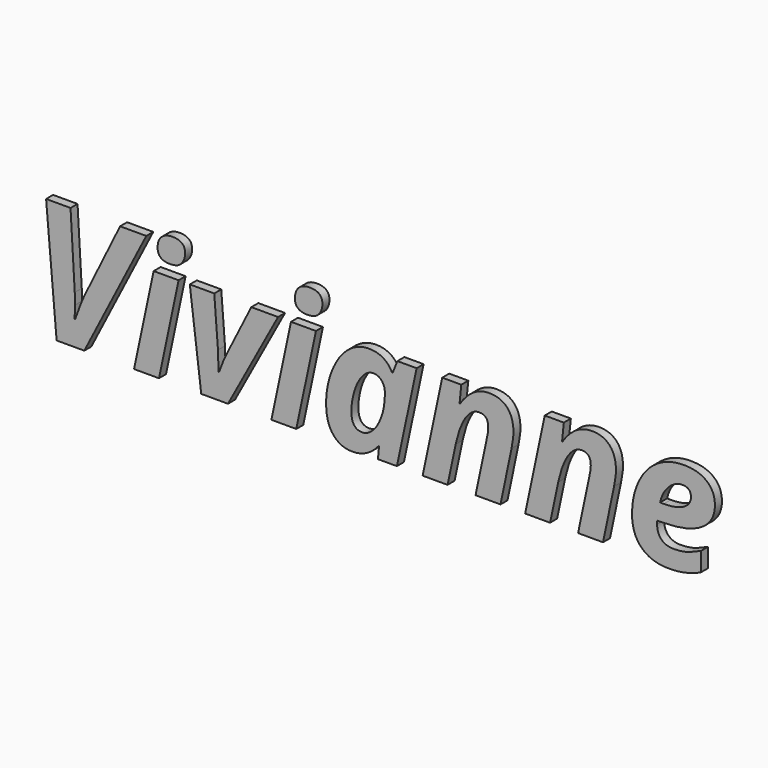
from build123d import *

# Parameters (mm, degrees)
F0_TEXT_SIZE = 61.4441750157
F1_DEPTH     = 3.175


# Not quite as in the source:
# - Text() gives the source's letters only with a copy of the font that has no kerning and outlines rounded to 1/6400 em; it was checked with that copy


with BuildPart() as f1:
    # F0 (on Front) → F1 (new body)
    with BuildSketch(Plane.XZ):
        with Locations((-54.9475252628, -63.2061734796)):
            Text('Vivianne', F0_TEXT_SIZE, font='Open Sans', font_style=FontStyle.BOLDITALIC, text_align=(TextAlign.LEFT, TextAlign.BOTTOM))
    extrude(amount=F1_DEPTH)


solid = f1.part
